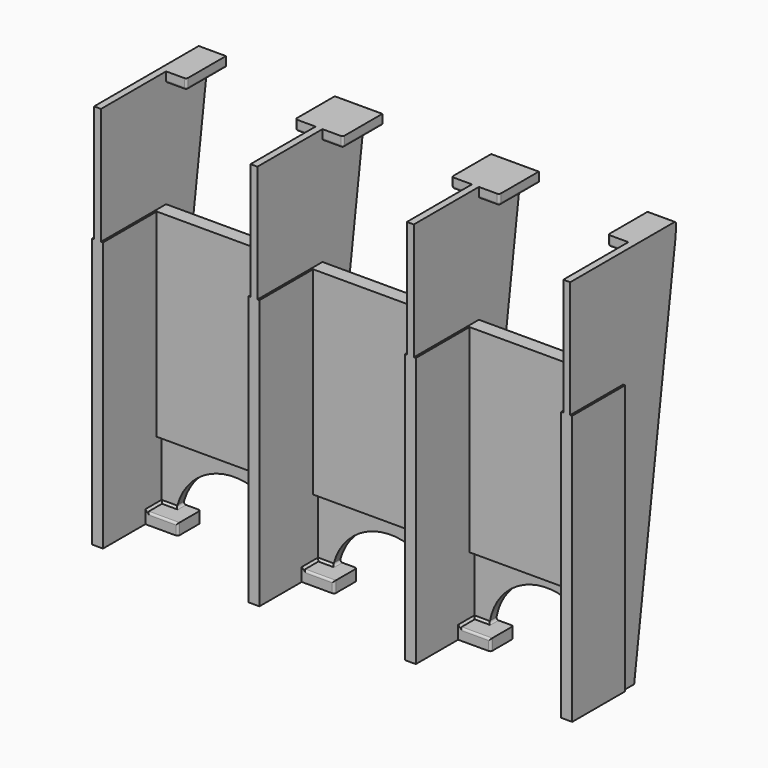
from build123d import *

# Parameters (mm, degrees)
F0_W           = 1
F0_H           = 32.5
F0_W_2         = 3.4
F0_H_2         = 0.5
F1_DEPTH       = 190
F2_DEPTH       = 57.5
F0_W_3         = 10
F0_H_3         = 25
F3_DEPTH       = 5
F4_DEPTH       = 57.5
F6_SIZE2       = 180
F6_SIZE        = 25
F7_W           = 71.5
F7_H           = 3
F8_DEPTH       = 35
F5_W           = 17
F5_H           = 5.5
F9_DEPTH       = 25
F12_DEPTH      = 25
F13_DEPTH      = 14
F14_DEPTH      = 11
F15_SIZE       = 1
F16_T1_DEPTH   = 4
F16_T6_DEPTH   = 4.2716810694
F16_T11_DEPTH  = 4.2716810694
F16_T16_DEPTH  = 4.2716810694
F16_T21_DEPTH  = 4.2716810694
F16_T26_DEPTH  = 3.9969928278
F16_T31_DEPTH  = 3.9969928278
F16_T33_DEPTH  = 10.5
F16_T35_DEPTH  = 191.7278184539
F16_T37_DEPTH  = 6.5
F16_T39_DEPTH  = 9
F16_T41_DEPTH  = 9
F16_T43_DEPTH  = 9
F16_T45_DEPTH  = 9
F16_T47_DEPTH  = 9
F16_T49_DEPTH  = 9
F16_T51_DEPTH  = 10
F16_T53_DEPTH  = 26.5
F16_T55_DEPTH  = 18.4
F16_T57_DEPTH  = 28.4
F16_T59_DEPTH  = 28.4
F16_T61_DEPTH  = 18.4
F16_S65_W      = 1
F16_S65_H      = 1
F16_T66_DEPTH  = 1
F16_S71_W      = 1
F16_S71_H      = 1
F16_T72_DEPTH  = 1
F16_S77_W      = 1
F16_S77_H      = 1
F16_T78_DEPTH  = 1
F16_S83_W      = 1
F16_S83_H      = 1
F16_T84_DEPTH  = 1
F16_S89_W      = 1
F16_S89_H      = 1
F16_T90_DEPTH  = 1
F16_S95_W      = 1
F16_S95_H      = 1
F16_T96_DEPTH  = 1
F16_T102_DEPTH = 20
F16_T107_DEPTH = 20
F16_T112_DEPTH = 20
F16_T117_DEPTH = 20
F16_T122_DEPTH = 20
F16_T127_DEPTH = 20


# Not quite as in the source:
# - a fillet or chamfer that OpenCascade refuses, or shapes differently, is made with other operations: its cross-section is extruded or revolved along the edge and cut away or added
# - a feature names something its author has since deleted; it is built from what else it names


with BuildPart() as f1:
    # F0 (on Top) → F1 (new body)
    with BuildSketch(Plane.XY):
        with Locations((-40.65, -18.75)):
            Rectangle(F0_W, F0_H)
        with Locations((36.25, -18.75)):
            Rectangle(F0_W, F0_H)
        with Locations((-113.15, -18.75)):
            Rectangle(F0_W, F0_H)
        with Locations((113.15, -18.75)):
            Rectangle(F0_W, F0_H)
        with Locations((38.45, -18.75)):
            Rectangle(F0_W_2, F0_H)
        with Locations((40.65, -18.75)):
            Rectangle(F0_W, F0_H)
        Polygon((36.75, -2.5), (40.15, -2.5), (40.15, -2), (40.15, 5), (40.15, 30), (36.75, 30), (36.75, 5), (36.75, -2), align=None)
        with Locations((115.35, -18.75)):
            Rectangle(F0_W_2, F0_H)
        Polygon((113.65, -2.5), (117.05, -2.5), (117.05, 30), (113.65, 30), (113.65, 5), (113.65, -2), align=None)
        with Locations((117.55, -18.75)):
            Rectangle(F0_W, F0_H)
        Polygon((-113.65, 30), (-117.05, 30), (-117.05, -2.5), (-117.05, -35), (-113.65, -35), (-113.65, -2.5), (-113.65, -2), (-113.65, 5), align=None)
        with Locations((-117.55, -18.75)):
            Rectangle(F0_W, F0_H)
        Polygon((-40.15, -35), (-36.75, -35), (-36.75, -2.5), (-36.75, -2), (-36.75, 5), (-36.75, 30), (-40.15, 30), (-40.15, 5), (-40.15, -2), (-40.15, -2.5), align=None)
        with Locations((-36.25, -18.75)):
            Rectangle(F0_W, F0_H)
        Polygon((35.75, -2), (36.75, -2), (36.75, 5), (26.75, 5), (-26.75, 5), (-36.75, 5), (-36.75, -2), (-35.75, -2), align=None)
        Polygon((-103.65, 5), (-113.65, 5), (-113.65, -2), (-112.65, -2), (-41.15, -2), (-40.15, -2), (-40.15, 5), (-50.15, 5), align=None)
        Polygon((112.65, -2), (113.65, -2), (113.65, 5), (103.65, 5), (50.15, 5), (40.15, 5), (40.15, -2), (41.15, -2), align=None)
        with Locations((-113.15, -2.25)):
            Rectangle(F0_W, F0_H_2)
        with Locations((-40.65, -2.25)):
            Rectangle(F0_W, F0_H_2)
        with Locations((-36.25, -2.25)):
            Rectangle(F0_W, F0_H_2)
        with Locations((36.25, -2.25)):
            Rectangle(F0_W, F0_H_2)
        with Locations((40.65, -2.25)):
            Rectangle(F0_W, F0_H_2)
        with Locations((113.15, -2.25)):
            Rectangle(F0_W, F0_H_2)
    extrude(amount=-F1_DEPTH)

    # F0 (on Top) → F2 (cut)
    with BuildSketch(Plane.XY):
        with Locations((-117.55, -18.75)):
            Rectangle(F0_W, F0_H)
        with Locations((-113.15, -18.75)):
            Rectangle(F0_W, F0_H)
        with Locations((-40.65, -18.75)):
            Rectangle(F0_W, F0_H)
        with Locations((-36.25, -18.75)):
            Rectangle(F0_W, F0_H)
        with Locations((36.25, -18.75)):
            Rectangle(F0_W, F0_H)
        with Locations((40.65, -18.75)):
            Rectangle(F0_W, F0_H)
        with Locations((113.15, -18.75)):
            Rectangle(F0_W, F0_H)
        with Locations((117.55, -18.75)):
            Rectangle(F0_W, F0_H)
        with Locations((113.15, -2.25)):
            Rectangle(F0_W, F0_H_2)
        with Locations((36.25, -2.25)):
            Rectangle(F0_W, F0_H_2)
        with Locations((40.65, -2.25)):
            Rectangle(F0_W, F0_H_2)
        with Locations((-36.25, -2.25)):
            Rectangle(F0_W, F0_H_2)
        with Locations((-40.65, -2.25)):
            Rectangle(F0_W, F0_H_2)
        with Locations((-113.15, -2.25)):
            Rectangle(F0_W, F0_H_2)
    extrude(amount=-F2_DEPTH, mode=Mode.SUBTRACT)

    # F0 (on Top) → F3 (join)
    with BuildSketch(Plane.XY):
        with Locations((108.65, 17.5)):
            Rectangle(F0_W_3, F0_H_3)
        with Locations((31.75, 17.5)):
            Rectangle(F0_W_3, F0_H_3)
        with Locations((-45.15, 17.5)):
            Rectangle(F0_W_3, F0_H_3)
        with Locations((-108.65, 17.5)):
            Rectangle(F0_W_3, F0_H_3)
        with Locations((-31.75, 17.5)):
            Rectangle(F0_W_3, F0_H_3)
        with Locations((45.15, 17.5)):
            Rectangle(F0_W_3, F0_H_3)
    extrude(amount=-F3_DEPTH)

    # F0 (on Top) → F4 (cut)
    with BuildSketch(Plane.XY):
        Polygon((-103.65, 5), (-113.65, 5), (-113.65, -2), (-112.65, -2), (-41.15, -2), (-40.15, -2), (-40.15, 5), (-50.15, 5), align=None)
        Polygon((35.75, -2), (36.75, -2), (36.75, 5), (26.75, 5), (-26.75, 5), (-36.75, 5), (-36.75, -2), (-35.75, -2), align=None)
        Polygon((112.65, -2), (113.65, -2), (113.65, 5), (103.65, 5), (50.15, 5), (40.15, 5), (40.15, -2), (41.15, -2), align=None)
    extrude(amount=-F4_DEPTH, mode=Mode.SUBTRACT)

    # F6
    f6_edges = [f1.edges().sort_by_distance(p)[0] for p in [
        (115.35, 30, -190),
        (38.45, 30, -190),
        (-38.45, 30, -190),
        (-115.35, 30, -190),
    ]]
    f6_side = f1.faces().sort_by_distance((0, -1.775321, -190))[0]
    chamfer(f6_edges, length=F6_SIZE, length2=F6_SIZE2, reference=f6_side)

    # F7 (on face) → F8 (cut)
    with BuildSketch(Plane(origin=(0, 0, -190), x_dir=(1, 0, 0), z_dir=(0, 0, -1))):
        with Locations((76.9, 0.5)):
            Rectangle(F7_W, F7_H)
        with Locations((0, 0.5)):
            Rectangle(F7_W, F7_H)
        with Locations((-76.9, 0.5)):
            Rectangle(F7_W, F7_H)
    extrude(amount=-F8_DEPTH, mode=Mode.SUBTRACT)

    # F5 (on face) → F9 (cut)
    with BuildSketch(Plane(origin=(0, 5, 0), x_dir=(-1, 0, 0), z_dir=(0, 1, 0))):
        with BuildLine():
            Line((-19.75, -184.5), (-19.75, -190))
            Line((-19.75, -190), (19.75, -190))
            Line((19.75, -190), (19.75, -184.5))
            Line((19.75, -184.5), (28.25, -184.5))
            ThreePointArc((28.25, -184.5), (0, -162.0193661972), (-28.25, -184.5))
            Line((-28.25, -184.5), (-19.75, -184.5))
        make_face()
        with Locations((-48.65, -187.25)):
            Rectangle(F5_W, F5_H)
        with Locations((-105.15, -187.25)):
            Rectangle(F5_W, F5_H)
        with Locations((48.65, -187.25)):
            Rectangle(F5_W, F5_H)
        with Locations((105.15, -187.25)):
            Rectangle(F5_W, F5_H)
        Polygon((-36.75, -184.5), (-36.75, -190), (-19.75, -190), (-19.75, -184.5), (-28.25, -184.5), align=None)
        Polygon((19.75, -184.5), (19.75, -190), (36.75, -190), (36.75, -184.5), (28.25, -184.5), align=None)
    extrude(amount=-F9_DEPTH, mode=Mode.SUBTRACT)

    # F11 (on face) + F10 (on face) → F12 (cut)
    with BuildSketch(Plane(origin=(0, 5, 0), x_dir=(-1, 0, 0), z_dir=(0, 1, 0))):
        with BuildLine():
            Line((96.65, -184.5), (105.15, -184.5))
            ThreePointArc((105.15, -184.5), (76.9, -162.0193661972), (48.65, -184.5))
            Line((48.65, -184.5), (57.15, -184.5))
            Line((57.15, -184.5), (57.15, -190))
            Line((57.15, -190), (96.65, -190))
            Line((96.65, -190), (96.65, -184.5))
        make_face()
    with BuildSketch(Plane(origin=(0, 5, 0), x_dir=(-1, 0, 0), z_dir=(0, 1, 0))):
        with BuildLine():
            Line((-57.15, -184.5), (-48.65, -184.5))
            ThreePointArc((-48.65, -184.5), (-76.9, -160), (-105.15, -184.5))
            Line((-105.15, -184.5), (-96.65, -184.5))
            Line((-96.65, -184.5), (-96.65, -190))
            Line((-96.65, -190), (-57.15, -190))
            Line((-57.15, -190), (-57.15, -184.5))
        make_face()
    extrude(amount=-F12_DEPTH, mode=Mode.SUBTRACT)

    # F5 (on face) → F13 (join)
    with BuildSketch(Plane(origin=(0, 5, 0), x_dir=(-1, 0, 0), z_dir=(0, 1, 0))):
        with Locations((-105.15, -187.25)):
            Rectangle(F5_W, F5_H)
        with Locations((-48.65, -187.25)):
            Rectangle(F5_W, F5_H)
        Polygon((-36.75, -184.5), (-36.75, -190), (-19.75, -190), (-19.75, -184.5), (-28.25, -184.5), align=None)
        Polygon((19.75, -184.5), (19.75, -190), (36.75, -190), (36.75, -184.5), (28.25, -184.5), align=None)
        with Locations((48.65, -187.25)):
            Rectangle(F5_W, F5_H)
        with Locations((105.15, -187.25)):
            Rectangle(F5_W, F5_H)
    extrude(amount=-F13_DEPTH)

    # F14 (add, through all): faces of the model
    f14_faces = [f1.faces().sort_by_distance(p)[0] for p in [
        (113.15, -20, -187.25),
        (40.65, -20, -187.25),
        (36.25, -20, -187.25),
        (-40.65, -20, -187.25),
        (-36.25, -20, -187.25),
        (-113.15, -20, -187.25),
    ]]
    extrude(f14_faces, amount=F14_DEPTH)

    # F15
    f15_edges = [f1.edges().sort_by_distance(p)[0] for p in [
        (112.65, -4, -184.5),
        (108.9, 1, -184.5),
        (44.9, 1, -184.5),
        (41.15, -4, -184.5),
        (32, 1, -184.5),
        (35.75, -4, -184.5),
        (-32, 1, -184.5),
        (-35.75, -4, -184.5),
        (-41.15, -4, -184.5),
        (-44.9, 1, -184.5),
        (-108.9, 1, -184.5),
        (-112.65, -4, -184.5),
    ]]
    chamfer(f15_edges, length=F15_SIZE)

    # F16: fillet of radius 1 on 54 edges, made by hand

    # F16_s2 → F16_t1 (join)
    with BuildSketch(Plane.XZ.offset(-5)):
        with BuildLine():
            ThreePointArc((103.9723944419, -184.5), (104.7414579069, -184.1391724234), (104.9555227592, -183.3170827736))
            ThreePointArc((104.9555227592, -183.3170827736), (105.0589736423, -183.9075200612), (105.15, -184.5))
            Line((105.15, -184.5), (103.9723944419, -184.5))
        make_face()
        with BuildLine():
            ThreePointArc((49.8276055581, -184.5), (49.0585420931, -184.1391724234), (48.8444772408, -183.3170827736))
            ThreePointArc((48.8444772408, -183.3170827736), (48.7410263577, -183.9075200612), (48.65, -184.5))
            Line((48.65, -184.5), (49.8276055581, -184.5))
        make_face()
        with BuildLine():
            ThreePointArc((-27.9274330911, -183.2317042488), (-27.7604305215, -184.1048571107), (-26.9640964989, -184.5))
            Line((-26.9640964989, -184.5), (-28.25, -184.5))
            ThreePointArc((-28.25, -184.5), (-28.0958740868, -183.8640317399), (-27.9274330911, -183.2317042488))
        make_face()
        with BuildLine():
            ThreePointArc((26.9640964989, -184.5), (27.7604305215, -184.1048571107), (27.9274330911, -183.2317042488))
            ThreePointArc((27.9274330911, -183.2317042488), (28.0958740868, -183.8640317399), (28.25, -184.5))
            Line((28.25, -184.5), (26.9640964989, -184.5))
        make_face()
        with BuildLine():
            ThreePointArc((-48.9725669089, -183.2317042488), (-49.1395694785, -184.1048571107), (-49.9359035011, -184.5))
            Line((-49.9359035011, -184.5), (-48.65, -184.5))
            ThreePointArc((-48.65, -184.5), (-48.8041259132, -183.8640317399), (-48.9725669089, -183.2317042488))
        make_face()
        with BuildLine():
            ThreePointArc((-103.8640964989, -184.5), (-104.6604305215, -184.1048571107), (-104.8274330911, -183.2317042488))
            ThreePointArc((-104.8274330911, -183.2317042488), (-104.9958740868, -183.8640317399), (-105.15, -184.5))
            Line((-105.15, -184.5), (-103.8640964989, -184.5))
        make_face()
    extrude(amount=F16_T1_DEPTH)


with BuildPart() as f16_tool4:
    # F16_s5 → F16_t6 (new body)
    with BuildSketch(Plane.XZ.offset(-1)):
        with BuildLine():
            ThreePointArc((-103.8640964989, -184.5), (-104.6604305215, -184.1048571107), (-104.8274330911, -183.2317042488))
            ThreePointArc((-104.8274330911, -183.2317042488), (-104.9958740868, -183.8640317399), (-105.15, -184.5))
            Line((-105.15, -184.5), (-103.8640964989, -184.5))
        make_face()
    extrude(amount=F16_T6_DEPTH)

    split(bisect_by=Plane(origin=(0, 92.25, -92.25), x_dir=(1, 0, 0), z_dir=(0, 0.7071067812, -0.7071067812)), keep=Keep.TOP)


with BuildPart() as f1_1:
    add(f1.part)

    # F16_t3: union F16_tool4
    add(f16_tool4.part)


with BuildPart() as f16_tool9:
    # F16_s10 → F16_t11 (new body)
    with BuildSketch(Plane.XZ.offset(-1)):
        with BuildLine():
            ThreePointArc((-48.9725669089, -183.2317042488), (-49.1395694785, -184.1048571107), (-49.9359035011, -184.5))
            Line((-49.9359035011, -184.5), (-48.65, -184.5))
            ThreePointArc((-48.65, -184.5), (-48.8041259132, -183.8640317399), (-48.9725669089, -183.2317042488))
        make_face()
    extrude(amount=F16_T11_DEPTH)

    split(bisect_by=Plane(origin=(0, 92.25, -92.25), x_dir=(1, 0, 0), z_dir=(0, 0.7071067812, -0.7071067812)), keep=Keep.TOP)


with BuildPart() as f1_2:
    add(f1_1.part)

    # F16_t8: union F16_tool9
    add(f16_tool9.part)


with BuildPart() as f16_tool14:
    # F16_s15 → F16_t16 (new body)
    with BuildSketch(Plane.XZ.offset(-1)):
        with BuildLine():
            ThreePointArc((26.9640964989, -184.5), (27.7604305215, -184.1048571107), (27.9274330911, -183.2317042488))
            ThreePointArc((27.9274330911, -183.2317042488), (28.0958740868, -183.8640317399), (28.25, -184.5))
            Line((28.25, -184.5), (26.9640964989, -184.5))
        make_face()
    extrude(amount=F16_T16_DEPTH)

    split(bisect_by=Plane(origin=(0, 92.25, -92.25), x_dir=(1, 0, 0), z_dir=(0, 0.7071067812, -0.7071067812)), keep=Keep.TOP)


with BuildPart() as f1_3:
    add(f1_2.part)

    # F16_t13: union F16_tool14
    add(f16_tool14.part)


with BuildPart() as f16_tool19:
    # F16_s20 → F16_t21 (new body)
    with BuildSketch(Plane.XZ.offset(-1)):
        with BuildLine():
            ThreePointArc((-27.9274330911, -183.2317042488), (-27.7604305215, -184.1048571107), (-26.9640964989, -184.5))
            Line((-26.9640964989, -184.5), (-28.25, -184.5))
            ThreePointArc((-28.25, -184.5), (-28.0958740868, -183.8640317399), (-27.9274330911, -183.2317042488))
        make_face()
    extrude(amount=F16_T21_DEPTH)

    split(bisect_by=Plane(origin=(0, 92.25, -92.25), x_dir=(1, 0, 0), z_dir=(0, 0.7071067812, -0.7071067812)), keep=Keep.TOP)


with BuildPart() as f1_4:
    add(f1_3.part)

    # F16_t18: union F16_tool19
    add(f16_tool19.part)


with BuildPart() as f16_tool24:
    # F16_s25 → F16_t26 (new body)
    with BuildSketch(Plane.XZ.offset(-1)):
        with BuildLine():
            ThreePointArc((49.8276055581, -184.5), (49.0585420931, -184.1391724234), (48.8444772408, -183.3170827736))
            ThreePointArc((48.8444772408, -183.3170827736), (48.7410263577, -183.9075200612), (48.65, -184.5))
            Line((48.65, -184.5), (49.8276055581, -184.5))
        make_face()
    extrude(amount=F16_T26_DEPTH)

    split(bisect_by=Plane(origin=(0, 92.25, -92.25), x_dir=(1, 0, 0), z_dir=(0, 0.7071067812, -0.7071067812)), keep=Keep.TOP)


with BuildPart() as f1_5:
    add(f1_4.part)

    # F16_t23: union F16_tool24
    add(f16_tool24.part)


with BuildPart() as f16_tool29:
    # F16_s30 → F16_t31 (new body)
    with BuildSketch(Plane.XZ.offset(-1)):
        with BuildLine():
            ThreePointArc((103.9723944419, -184.5), (104.7414579069, -184.1391724234), (104.9555227592, -183.3170827736))
            ThreePointArc((104.9555227592, -183.3170827736), (105.0589736423, -183.9075200612), (105.15, -184.5))
            Line((105.15, -184.5), (103.9723944419, -184.5))
        make_face()
    extrude(amount=F16_T31_DEPTH)

    split(bisect_by=Plane(origin=(0, 92.25, -92.25), x_dir=(1, 0, 0), z_dir=(0, 0.7071067812, -0.7071067812)), keep=Keep.TOP)


with BuildPart() as f1_6:
    add(f1_5.part)

    # F16_t28: union F16_tool29
    add(f16_tool29.part)

    # F16_s34 → F16_t33 (cut)
    with BuildSketch(Plane.XY.offset(-192.5)):
        with BuildLine():
            ThreePointArc((56.15, -9), (56.8571067812, -8.7071067812), (57.15, -8))
            Line((57.15, -8), (57.15, -9))
            Line((57.15, -9), (56.15, -9))
        make_face()
        with BuildLine():
            ThreePointArc((20.75, -9), (20.0428932188, -8.7071067812), (19.75, -8))
            Line((19.75, -8), (19.75, -9))
            Line((19.75, -9), (20.75, -9))
        make_face()
        with BuildLine():
            ThreePointArc((97.65, -9), (96.9428932188, -8.7071067812), (96.65, -8))
            Line((96.65, -8), (96.65, -9))
            Line((96.65, -9), (97.65, -9))
        make_face()
        with BuildLine():
            ThreePointArc((-20.75, -9), (-20.0428932188, -8.7071067812), (-19.75, -8))
            Line((-19.75, -8), (-19.75, -9))
            Line((-19.75, -9), (-20.75, -9))
        make_face()
        with BuildLine():
            ThreePointArc((-57.15, -8), (-56.8571067812, -8.7071067812), (-56.15, -9))
            Line((-56.15, -9), (-57.15, -9))
            Line((-57.15, -9), (-57.15, -8))
        make_face()
        with BuildLine():
            ThreePointArc((-96.65, -8), (-96.9428932188, -8.7071067812), (-97.65, -9))
            Line((-97.65, -9), (-96.65, -9))
            Line((-96.65, -9), (-96.65, -8))
        make_face()
        with BuildLine():
            ThreePointArc((-57.15, 4), (-56.8571067812, 4.7071067812), (-56.15, 5))
            Line((-56.15, 5), (-57.15, 5))
            Line((-57.15, 5), (-57.15, 4))
        make_face()
        with BuildLine():
            ThreePointArc((-19.75, 4), (-20.0428932188, 4.7071067812), (-20.75, 5))
            Line((-20.75, 5), (-19.75, 5))
            Line((-19.75, 5), (-19.75, 4))
        make_face()
        with BuildLine():
            ThreePointArc((19.75, 4), (20.0428932188, 4.7071067812), (20.75, 5))
            Line((20.75, 5), (19.75, 5))
            Line((19.75, 5), (19.75, 4))
        make_face()
        with BuildLine():
            ThreePointArc((56.15, 5), (56.8571067812, 4.7071067812), (57.15, 4))
            Line((57.15, 4), (57.15, 5))
            Line((57.15, 5), (56.15, 5))
        make_face()
        with BuildLine():
            ThreePointArc((97.65, 5), (96.9428932188, 4.7071067812), (96.65, 4))
            Line((96.65, 4), (96.65, 5))
            Line((96.65, 5), (97.65, 5))
        make_face()
        with BuildLine():
            ThreePointArc((-97.65, 5), (-96.9428932188, 4.7071067812), (-96.65, 4))
            Line((-96.65, 4), (-96.65, 5))
            Line((-96.65, 5), (-97.65, 5))
        make_face()
    extrude(amount=F16_T33_DEPTH, mode=Mode.SUBTRACT)

    # F16_s36 → F16_t35 (cut)
    with BuildSketch(Plane(origin=(0, -26.1387733127, -188.1991678518), x_dir=(1, 0, 0), z_dir=(0, 0.1375683713, 0.9904922732))):
        with BuildLine():
            ThreePointArc((-116.05, 31.0904519081), (-116.7571067812, 30.7975586893), (-117.05, 30.0904519081))
            Line((-117.05, 30.0904519081), (-117.05, 31.0904519081))
            Line((-117.05, 31.0904519081), (-116.05, 31.0904519081))
        make_face()
        with BuildLine():
            ThreePointArc((117.05, 30.0904519081), (116.7571067812, 30.7975586893), (116.05, 31.0904519081))
            Line((116.05, 31.0904519081), (117.05, 31.0904519081))
            Line((117.05, 31.0904519081), (117.05, 30.0904519081))
        make_face()
    extrude(amount=F16_T35_DEPTH, mode=Mode.SUBTRACT)

    # F16_s38 → F16_t37 (cut)
    with BuildSketch(Plane.XY.offset(-4)):
        with BuildLine():
            ThreePointArc((50.15, 6), (49.8571067812, 5.2928932188), (49.15, 5))
            Line((49.15, 5), (50.15, 5))
            Line((50.15, 5), (50.15, 6))
        make_face()
        with BuildLine():
            ThreePointArc((26.75, 6), (27.0428932188, 5.2928932188), (27.75, 5))
            Line((27.75, 5), (26.75, 5))
            Line((26.75, 5), (26.75, 6))
        make_face()
        with BuildLine():
            ThreePointArc((104.65, 5), (103.9428932188, 5.2928932188), (103.65, 6))
            Line((103.65, 6), (103.65, 5))
            Line((103.65, 5), (104.65, 5))
        make_face()
        with BuildLine():
            ThreePointArc((-26.75, 6), (-27.0428932188, 5.2928932188), (-27.75, 5))
            Line((-27.75, 5), (-26.75, 5))
            Line((-26.75, 5), (-26.75, 6))
        make_face()
        with BuildLine():
            ThreePointArc((-50.15, 6), (-49.8571067812, 5.2928932188), (-49.15, 5))
            Line((-49.15, 5), (-50.15, 5))
            Line((-50.15, 5), (-50.15, 6))
        make_face()
        with BuildLine():
            ThreePointArc((-103.65, 6), (-103.9428932188, 5.2928932188), (-104.65, 5))
            Line((-104.65, 5), (-103.65, 5))
            Line((-103.65, 5), (-103.65, 6))
        make_face()
    extrude(amount=F16_T37_DEPTH, mode=Mode.SUBTRACT)

    # F16_s40 → F16_t39 (cut)
    with BuildSketch(Plane.YZ.offset(104.65)):
        with BuildLine():
            ThreePointArc((6, -5), (5.2928932188, -4.7071067812), (5, -4))
            Line((5, -4), (5, -5))
            Line((5, -5), (6, -5))
        make_face()
    extrude(amount=F16_T39_DEPTH, mode=Mode.SUBTRACT)

    # F16_s42 → F16_t41 (cut)
    with BuildSketch(Plane.YZ.offset(40.15)):
        with BuildLine():
            ThreePointArc((6, -5), (5.2928932188, -4.7071067812), (5, -4))
            Line((5, -4), (5, -5))
            Line((5, -5), (6, -5))
        make_face()
    extrude(amount=F16_T41_DEPTH, mode=Mode.SUBTRACT)

    # F16_s44 → F16_t43 (cut)
    with BuildSketch(Plane.YZ.offset(27.75)):
        with BuildLine():
            ThreePointArc((6, -5), (5.2928932188, -4.7071067812), (5, -4))
            Line((5, -4), (5, -5))
            Line((5, -5), (6, -5))
        make_face()
    extrude(amount=F16_T43_DEPTH, mode=Mode.SUBTRACT)

    # F16_s46 → F16_t45 (cut)
    with BuildSketch(Plane.YZ.offset(-36.75)):
        with BuildLine():
            ThreePointArc((6, -5), (5.2928932188, -4.7071067812), (5, -4))
            Line((5, -4), (5, -5))
            Line((5, -5), (6, -5))
        make_face()
    extrude(amount=F16_T45_DEPTH, mode=Mode.SUBTRACT)

    # F16_s48 → F16_t47 (cut)
    with BuildSketch(Plane.YZ.offset(-49.15)):
        with BuildLine():
            ThreePointArc((5, -4), (5.2928932188, -4.7071067812), (6, -5))
            Line((6, -5), (5, -5))
            Line((5, -5), (5, -4))
        make_face()
    extrude(amount=F16_T47_DEPTH, mode=Mode.SUBTRACT)

    # F16_s50 → F16_t49 (cut)
    with BuildSketch(Plane.YZ.offset(-113.65)):
        with BuildLine():
            ThreePointArc((5, -4), (5.2928932188, -4.7071067812), (6, -5))
            Line((6, -5), (5, -5))
            Line((5, -5), (5, -4))
        make_face()
    extrude(amount=F16_T49_DEPTH, mode=Mode.SUBTRACT)

    # F16_s52 → F16_t51 (cut)
    with BuildSketch(Plane.XY.offset(-7.5)):
        with BuildLine():
            ThreePointArc((-104.65, 30), (-103.9428932188, 29.7071067812), (-103.65, 29))
            Line((-103.65, 29), (-103.65, 30))
            Line((-103.65, 30), (-104.65, 30))
        make_face()
        with BuildLine():
            ThreePointArc((-49.15, 30), (-49.8571067812, 29.7071067812), (-50.15, 29))
            Line((-50.15, 29), (-50.15, 30))
            Line((-50.15, 30), (-49.15, 30))
        make_face()
        with BuildLine():
            ThreePointArc((-26.75, 29), (-27.0428932188, 29.7071067812), (-27.75, 30))
            Line((-27.75, 30), (-26.75, 30))
            Line((-26.75, 30), (-26.75, 29))
        make_face()
        with BuildLine():
            ThreePointArc((26.75, 29), (27.0428932188, 29.7071067812), (27.75, 30))
            Line((27.75, 30), (26.75, 30))
            Line((26.75, 30), (26.75, 29))
        make_face()
        with BuildLine():
            ThreePointArc((50.15, 29), (49.8571067812, 29.7071067812), (49.15, 30))
            Line((49.15, 30), (50.15, 30))
            Line((50.15, 30), (50.15, 29))
        make_face()
        with BuildLine():
            ThreePointArc((104.65, 30), (103.9428932188, 29.7071067812), (103.65, 29))
            Line((103.65, 29), (103.65, 30))
            Line((103.65, 30), (104.65, 30))
        make_face()
    extrude(amount=F16_T51_DEPTH, mode=Mode.SUBTRACT)

    # F16_s54 → F16_t53 (cut)
    with BuildSketch(Plane.XZ.offset(-32.5)):
        with BuildLine():
            ThreePointArc((-103.65, -4), (-103.9428932188, -4.7071067812), (-104.65, -5))
            Line((-104.65, -5), (-103.65, -5))
            Line((-103.65, -5), (-103.65, -4))
        make_face()
        with BuildLine():
            ThreePointArc((-50.15, -4), (-49.8571067812, -4.7071067812), (-49.15, -5))
            Line((-49.15, -5), (-50.15, -5))
            Line((-50.15, -5), (-50.15, -4))
        make_face()
        with BuildLine():
            ThreePointArc((-27.75, -5), (-27.0428932188, -4.7071067812), (-26.75, -4))
            Line((-26.75, -4), (-26.75, -5))
            Line((-26.75, -5), (-27.75, -5))
        make_face()
        with BuildLine():
            ThreePointArc((27.75, -5), (27.0428932188, -4.7071067812), (26.75, -4))
            Line((26.75, -4), (26.75, -5))
            Line((26.75, -5), (27.75, -5))
        make_face()
        with BuildLine():
            ThreePointArc((50.15, -4), (49.8571067812, -4.7071067812), (49.15, -5))
            Line((49.15, -5), (50.15, -5))
            Line((50.15, -5), (50.15, -4))
        make_face()
        with BuildLine():
            ThreePointArc((104.65, -5), (103.9428932188, -4.7071067812), (103.65, -4))
            Line((103.65, -4), (103.65, -5))
            Line((103.65, -5), (104.65, -5))
        make_face()
    extrude(amount=F16_T53_DEPTH, mode=Mode.SUBTRACT)

    # F16_s56 → F16_t55 (cut)
    with BuildSketch(Plane.YZ.offset(101.15)):
        with BuildLine():
            ThreePointArc((30, -1), (29.7071067812, -0.2928932188), (29, 0))
            Line((29, 0), (30, 0))
            Line((30, 0), (30, -1))
        make_face()
    extrude(amount=F16_T55_DEPTH, mode=Mode.SUBTRACT)

    # F16_s58 → F16_t57 (cut)
    with BuildSketch(Plane.YZ.offset(24.25)):
        with BuildLine():
            ThreePointArc((29, 0), (29.7071067812, -0.2928932188), (30, -1))
            Line((30, -1), (30, 0))
            Line((30, 0), (29, 0))
        make_face()
    extrude(amount=F16_T57_DEPTH, mode=Mode.SUBTRACT)

    # F16_s60 → F16_t59 (cut)
    with BuildSketch(Plane.YZ.offset(-52.65)):
        with BuildLine():
            ThreePointArc((30, -1), (29.7071067812, -0.2928932188), (29, 0))
            Line((29, 0), (30, 0))
            Line((30, 0), (30, -1))
        make_face()
    extrude(amount=F16_T59_DEPTH, mode=Mode.SUBTRACT)

    # F16_s62 → F16_t61 (cut)
    with BuildSketch(Plane.YZ.offset(-119.55)):
        with BuildLine():
            ThreePointArc((30, -1), (29.7071067812, -0.2928932188), (29, 0))
            Line((29, 0), (30, 0))
            Line((30, 0), (30, -1))
        make_face()
    extrude(amount=F16_T61_DEPTH, mode=Mode.SUBTRACT)


with BuildPart() as f16_tool64:
    # F16_s65 → F16_t66 (new body)
    with BuildSketch(Plane.XZ.offset(-6)):
        with Locations((49.65, -4.5)):
            Rectangle(F16_S65_W, F16_S65_H)
    extrude(amount=F16_T66_DEPTH)

    # F16_s67 → F16_t68 (revolve, cut)
    with BuildSketch(Plane(origin=(49.15, 6, -4), x_dir=(-0.7071067812, 0, 0.7071067812), z_dir=(0.7071067812, 0, 0.7071067812))):
        with BuildLine():
            ThreePointArc((0, -1), (1, 0), (0, 1))
            Line((0, 1), (0, -1))
        make_face()
    revolve(axis=Axis((49.15, 6, -4), (0, -1, 0)), mode=Mode.SUBTRACT)


with BuildPart() as f1_7:
    add(f1_6.part)

    # F16_t63: cut F16_tool64
    add(f16_tool64.part, mode=Mode.SUBTRACT)


with BuildPart() as f16_tool70:
    # F16_s71 → F16_t72 (new body)
    with BuildSketch(Plane.XY.offset(-4)):
        with Locations((27.25, 5.5)):
            Rectangle(F16_S71_W, F16_S71_H)
    extrude(amount=-F16_T72_DEPTH)

    # F16_s73 → F16_t74 (revolve, cut)
    with BuildSketch(Plane(origin=(27.75, 6, -4), x_dir=(0.7071067812, 0.7071067812, 0), z_dir=(-0.7071067812, 0.7071067812, 0))):
        with BuildLine():
            ThreePointArc((0, -1), (1, 0), (0, 1))
            Line((0, 1), (0, -1))
        make_face()
    revolve(axis=Axis((27.75, 6, -4), (0, 0, -1)), mode=Mode.SUBTRACT)


with BuildPart() as f1_8:
    add(f1_7.part)

    # F16_t69: cut F16_tool70
    add(f16_tool70.part, mode=Mode.SUBTRACT)


with BuildPart() as f16_tool76:
    # F16_s77 → F16_t78 (new body)
    with BuildSketch(Plane.XY.offset(-4)):
        with Locations((104.15, 5.5)):
            Rectangle(F16_S77_W, F16_S77_H)
    extrude(amount=-F16_T78_DEPTH)

    # F16_s79 → F16_t80 (revolve, cut)
    with BuildSketch(Plane(origin=(104.65, 6, -4), x_dir=(0.7071067812, 0.7071067812, 0), z_dir=(-0.7071067812, 0.7071067812, 0))):
        with BuildLine():
            ThreePointArc((0, -1), (1, 0), (0, 1))
            Line((0, 1), (0, -1))
        make_face()
    revolve(axis=Axis((104.65, 6, -4), (0, 0, -1)), mode=Mode.SUBTRACT)


with BuildPart() as f1_9:
    add(f1_8.part)

    # F16_t75: cut F16_tool76
    add(f16_tool76.part, mode=Mode.SUBTRACT)


with BuildPart() as f16_tool82:
    # F16_s83 → F16_t84 (new body)
    with BuildSketch(Plane.YZ.offset(-27.75)):
        with Locations((5.5, -4.5)):
            Rectangle(F16_S83_W, F16_S83_H)
    extrude(amount=F16_T84_DEPTH)

    # F16_s85 → F16_t86 (revolve, cut)
    with BuildSketch(Plane(origin=(-27.75, 6, -4), x_dir=(0, 0.7071067812, 0.7071067812), z_dir=(0, 0.7071067812, -0.7071067812))):
        with BuildLine():
            ThreePointArc((0, -1), (1, 0), (0, 1))
            Line((0, 1), (0, -1))
        make_face()
    revolve(axis=Axis((-27.75, 6, -4), (1, 0, 0)), mode=Mode.SUBTRACT)


with BuildPart() as f1_10:
    add(f1_9.part)

    # F16_t81: cut F16_tool82
    add(f16_tool82.part, mode=Mode.SUBTRACT)


with BuildPart() as f16_tool88:
    # F16_s89 → F16_t90 (new body)
    with BuildSketch(Plane.YZ.offset(-49.15)):
        with Locations((5.5, -4.5)):
            Rectangle(F16_S89_W, F16_S89_H)
    extrude(amount=-F16_T90_DEPTH)

    # F16_s91 → F16_t92 (revolve, cut)
    with BuildSketch(Plane(origin=(-49.15, 6, -4), x_dir=(0, 0.7071067812, 0.7071067812), z_dir=(0, -0.7071067812, 0.7071067812))):
        with BuildLine():
            ThreePointArc((0, -1), (1, 0), (0, 1))
            Line((0, 1), (0, -1))
        make_face()
    revolve(axis=Axis((-49.15, 6, -4), (-1, 0, 0)), mode=Mode.SUBTRACT)


with BuildPart() as f1_11:
    add(f1_10.part)

    # F16_t87: cut F16_tool88
    add(f16_tool88.part, mode=Mode.SUBTRACT)


with BuildPart() as f16_tool94:
    # F16_s95 → F16_t96 (new body)
    with BuildSketch(Plane.YZ.offset(-104.65)):
        with Locations((5.5, -4.5)):
            Rectangle(F16_S95_W, F16_S95_H)
    extrude(amount=F16_T96_DEPTH)

    # F16_s97 → F16_t98 (revolve, cut)
    with BuildSketch(Plane(origin=(-104.65, 6, -4), x_dir=(0, 0.7071067812, 0.7071067812), z_dir=(0, 0.7071067812, -0.7071067812))):
        with BuildLine():
            ThreePointArc((0, -1), (1, 0), (0, 1))
            Line((0, 1), (0, -1))
        make_face()
    revolve(axis=Axis((-104.65, 6, -4), (1, 0, 0)), mode=Mode.SUBTRACT)


with BuildPart() as f1_12:
    add(f1_11.part)

    # F16_t93: cut F16_tool94
    add(f16_tool94.part, mode=Mode.SUBTRACT)


with BuildPart() as f16_tool100:
    # F16_s101 → F16_t102 (new body)
    with BuildSketch(Plane.YZ.offset(-114.15)):
        with BuildLine():
            ThreePointArc((-8, -184.5), (-8.7071067812, -184.7928932188), (-9, -185.5))
            Line((-9, -185.5), (-9, -184.5))
            Line((-9, -184.5), (-8, -184.5))
        make_face()
    extrude(amount=F16_T102_DEPTH)

    split(bisect_by=Plane(origin=(-148.075, 0, -148.075), x_dir=(0, 1, 0), z_dir=(0.7071067812, 0, 0.7071067812)), keep=Keep.TOP)


with BuildPart() as f1_13:
    add(f1_12.part)

    # F16_t99: cut F16_tool100
    add(f16_tool100.part, mode=Mode.SUBTRACT)


with BuildPart() as f16_tool105:
    # F16_s106 → F16_t107 (new body)
    with BuildSketch(Plane.YZ.offset(-59.65)):
        with BuildLine():
            ThreePointArc((-8, -184.5), (-8.7071067812, -184.7928932188), (-9, -185.5))
            Line((-9, -185.5), (-9, -184.5))
            Line((-9, -184.5), (-8, -184.5))
        make_face()
    extrude(amount=F16_T107_DEPTH)

    split(bisect_by=Plane(origin=(71.175, 0, -71.175), x_dir=(0, 1, 0), z_dir=(-0.7071067812, 0, 0.7071067812)), keep=Keep.TOP)


with BuildPart() as f1_14:
    add(f1_13.part)

    # F16_t104: cut F16_tool105
    add(f16_tool105.part, mode=Mode.SUBTRACT)


with BuildPart() as f16_tool110:
    # F16_s111 → F16_t112 (new body)
    with BuildSketch(Plane.YZ.offset(-37.25)):
        with BuildLine():
            ThreePointArc((-8, -184.5), (-8.7071067812, -184.7928932188), (-9, -185.5))
            Line((-9, -185.5), (-9, -184.5))
            Line((-9, -184.5), (-8, -184.5))
        make_face()
    extrude(amount=F16_T112_DEPTH)

    split(bisect_by=Plane(origin=(-109.625, 0, -109.625), x_dir=(0, 1, 0), z_dir=(0.7071067812, 0, 0.7071067812)), keep=Keep.TOP)


with BuildPart() as f1_15:
    add(f1_14.part)

    # F16_t109: cut F16_tool110
    add(f16_tool110.part, mode=Mode.SUBTRACT)


with BuildPart() as f16_tool115:
    # F16_s116 → F16_t117 (new body)
    with BuildSketch(Plane.YZ.offset(17.25)):
        with BuildLine():
            ThreePointArc((-9, -185.5), (-8.7071067812, -184.7928932188), (-8, -184.5))
            Line((-8, -184.5), (-9, -184.5))
            Line((-9, -184.5), (-9, -185.5))
        make_face()
    extrude(amount=F16_T117_DEPTH)

    split(bisect_by=Plane(origin=(109.625, 0, -109.625), x_dir=(0, 1, 0), z_dir=(-0.7071067812, 0, 0.7071067812)), keep=Keep.TOP)


with BuildPart() as f1_16:
    add(f1_15.part)

    # F16_t114: cut F16_tool115
    add(f16_tool115.part, mode=Mode.SUBTRACT)


with BuildPart() as f16_tool120:
    # F16_s121 → F16_t122 (new body)
    with BuildSketch(Plane.YZ.offset(39.65)):
        with BuildLine():
            ThreePointArc((-9, -185.5), (-8.7071067812, -184.7928932188), (-8, -184.5))
            Line((-8, -184.5), (-9, -184.5))
            Line((-9, -184.5), (-9, -185.5))
        make_face()
    extrude(amount=F16_T122_DEPTH)

    split(bisect_by=Plane(origin=(-71.175, 0, -71.175), x_dir=(0, 1, 0), z_dir=(0.7071067812, 0, 0.7071067812)), keep=Keep.TOP)


with BuildPart() as f1_17:
    add(f1_16.part)

    # F16_t119: cut F16_tool120
    add(f16_tool120.part, mode=Mode.SUBTRACT)


with BuildPart() as f16_tool125:
    # F16_s126 → F16_t127 (new body)
    with BuildSketch(Plane.YZ.offset(94.15)):
        with BuildLine():
            ThreePointArc((-9, -185.5), (-8.7071067812, -184.7928932188), (-8, -184.5))
            Line((-8, -184.5), (-9, -184.5))
            Line((-9, -184.5), (-9, -185.5))
        make_face()
    extrude(amount=F16_T127_DEPTH)

    split(bisect_by=Plane(origin=(148.075, 0, -148.075), x_dir=(0, 1, 0), z_dir=(-0.7071067812, 0, 0.7071067812)), keep=Keep.TOP)


with BuildPart() as f1_18:
    add(f1_17.part)

    # F16_t124: cut F16_tool125
    add(f16_tool125.part, mode=Mode.SUBTRACT)


solid = f1_18.part
